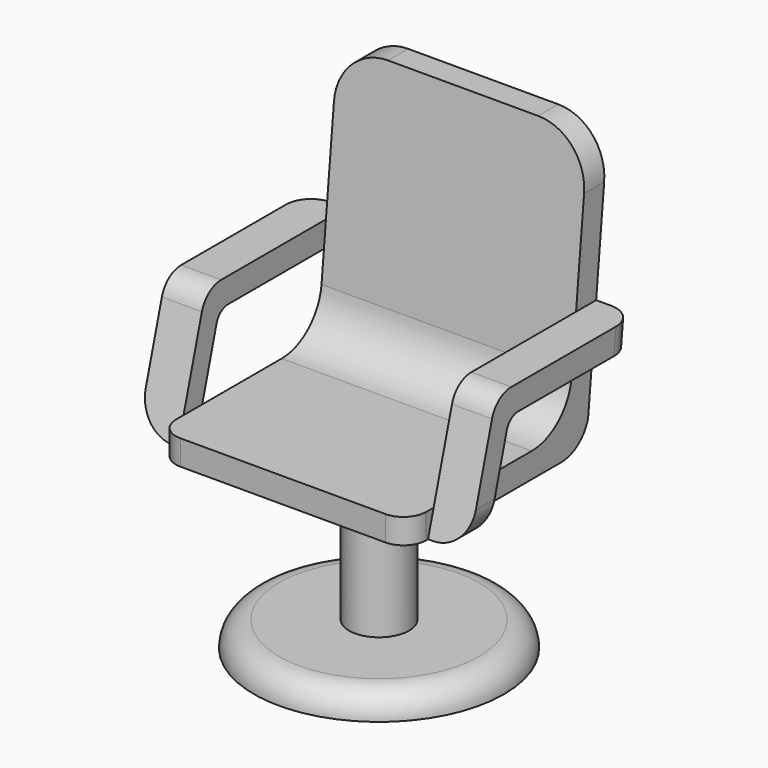
from build123d import *

# Parameters (mm, degrees)
F0_R         = 250
F1_DEPTH     = 50
F2_R         = 60
F3_DEPTH     = 300
F5_DEPTH     = 250
F7_DEPTH     = 80
F9_R         = 45
F10_R        = 100
F11_R        = 100
F12_T1_DEPTH = 835.410196625
F13_R        = 50
F14_R        = 30
F15_R        = 70
F16_R        = 50
F17_R        = 49.99999


# Not quite as in the source:
# - a fillet or chamfer that OpenCascade refuses, or shapes differently, is made with other operations: its cross-section is extruded or revolved along the edge and cut away or added
# - a fillet or chamfer is up to 0.001 mm smaller than in the source, because OpenCascade refuses the exact size


with BuildPart() as f1:
    # F0 (on Top) → F1 (new body)
    with BuildSketch(Plane.XY):
        Circle(F0_R)
    extrude(amount=F1_DEPTH)

    # F2 (on face) → F3 (join)
    with BuildSketch(Plane.XY.offset(50)):
        Circle(F2_R)
    extrude(amount=F3_DEPTH)

    # F17 (radius 50 in the source; OpenCascade refuses exactly that, so slightly less here)
    f17_edges = [f1.edges().sort_by_distance(p)[0] for p in [
        (-250, 0, 50),
    ]]
    fillet(f17_edges, radius=F17_R)


with BuildPart() as f5:
    # F4 (on Right) → F5 (new body, symmetric)
    with BuildSketch(Plane.YZ):
        Polygon((159.748109237, 400), (-240, 400), (-240, 350), (210, 350), (210, 400), (260.251890763, 900), (210, 900), align=None)
    extrude(amount=F5_DEPTH, both=True)

    # F6 (on face) → F7 (join)
    with BuildSketch(Plane.YZ.offset(250)):
        Polygon((225.0755672289, 550), (230.1007563052, 600), (179.8488655422, 600), (174.8236764659, 550), align=None)
        Polygon((-129.2442374825, 400), (-175.979848739, 400), (-190, 350), (-143.2643887435, 350), align=None)
        Polygon((174.8236764659, 550), (179.8488655422, 600), (-119.8992436948, 600), (-175.979848739, 400), (-129.2442374825, 400), (-87.1837836993, 550), align=None)
    extrude(amount=F7_DEPTH)

    # F8: F5 across plane


with BuildPart() as f5_1:
    add(f5.part)
    add(f5.part.mirror(Plane.YZ))

    # F9
    f9_edges = [f5_1.edges().sort_by_distance(p)[0] for p in [
        (250, -240, 375),
        (-250, -240, 375),
    ]]
    fillet(f9_edges, radius=F9_R)

    # F10
    f10_edges = [f5_1.edges().sort_by_distance(p)[0] for p in [
        (250, 235.125945, 900),
        (-250, 235.125945, 900),
    ]]
    fillet(f10_edges, radius=F10_R)

    # F11
    f11_edges = [f5_1.edges().sort_by_distance(p)[0] for p in [
        (0, 159.748109, 400),
    ]]
    fillet(f11_edges, radius=F11_R)

    # F12: fillet of radius 70 on 1 edges, made by hand

    # F12_s2 → F12_t1 (cut)
    with BuildSketch(Plane.YZ.offset(-417.7050983125)):
        with BuildLine():
            ThreePointArc((210, 400), (184.7509620017, 363.8751391984), (142.917960675, 350))
            Line((142.917960675, 350), (210, 350))
            Line((210, 350), (210, 400))
        make_face()
    extrude(amount=F12_T1_DEPTH, mode=Mode.SUBTRACT)

    # F13
    f13_edges = [f5_1.edges().sort_by_distance(p)[0] for p in [
        (290, -119.899244, 600),
        (-290, -119.899244, 600),
    ]]
    fillet(f13_edges, radius=F13_R)

    # F14
    f14_edges = [f5_1.edges().sort_by_distance(p)[0] for p in [
        (290, -87.183784, 550),
        (-290, -87.183784, 550),
    ]]
    fillet(f14_edges, radius=F14_R)

    # F15
    f15_edges = [f5_1.edges().sort_by_distance(p)[0] for p in [
        (330, -166.632194, 350),
        (-330, -166.632194, 350),
    ]]
    fillet(f15_edges, radius=F15_R)

    # F16
    f16_edges = [f5_1.edges().sort_by_distance(p)[0] for p in [
        (330, 227.588162, 575),
        (-330, 227.588162, 575),
    ]]
    fillet(f16_edges, radius=F16_R)


solid = Compound([f1.part, f5_1.part])
